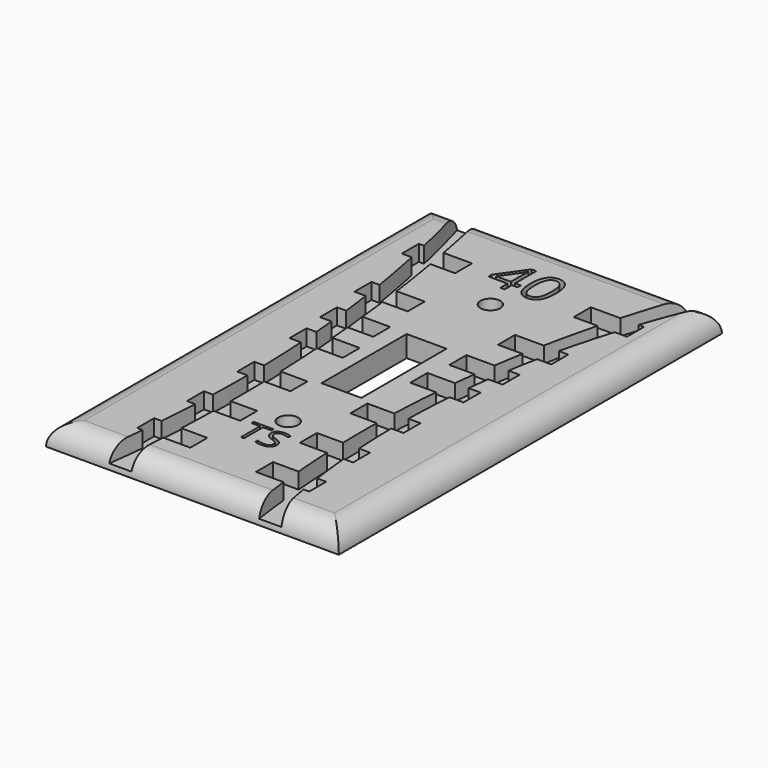
from build123d import *

# Parameters (mm, degrees)
F1_DEPTH     = 5.08
F4_R         = 5.07999
F2_TEXT_SIZE = 8.8219803325
F3_TEXT_SIZE = 13.1538772758
F5_DEPTH     = 3.81


# Not quite as in the source:
# - a fillet or chamfer is up to 0.001 mm smaller than in the source, because OpenCascade refuses the exact size
# - Text() gives the source's letters only with a copy of the font that has no kerning and outlines rounded to 1/6400 em; it was checked with that copy


with BuildPart() as f1:
    # F0 (on Top) → F1 (new body)
    with BuildSketch(Plane.XY):
        with BuildLine():
            Line((0, 34.13125), (0, 57.15))
            Line((0, 57.15), (-34.925, 57.15))
            Line((-34.925, 57.15), (-34.925, 0))
            Line((-34.925, 0), (-4.7625, 0))
            Line((-4.7625, 0), (-4.7625, 12.7))
            Line((-4.7625, 12.7), (0, 12.7))
            Line((0, 12.7), (0, 29.36875))
            ThreePointArc((0, 29.36875), (-2.38125, 31.75), (0, 34.13125))
        make_face()
        with BuildLine():
            Line((34.925, 57.15), (0, 57.15))
            Line((0, 57.15), (0, 34.13125))
            ThreePointArc((0, 34.13125), (1.6837980227, 33.4337980227), (2.38125, 31.75))
            ThreePointArc((2.38125, 31.75), (1.6837980227, 30.0662019773), (0, 29.36875))
            Line((0, 29.36875), (0, 12.7))
            Line((0, 12.7), (4.7625, 12.7))
            Line((4.7625, 12.7), (4.7625, 0))
            Line((4.7625, 0), (34.925, 0))
            Line((34.925, 0), (34.925, 57.15))
        make_face()
        with BuildLine():
            Line((-4.7625, 0), (-34.925, 0))
            Line((-34.925, 0), (-34.925, -57.15))
            Line((-34.925, -57.15), (0, -57.15))
            Line((0, -57.15), (0, -30.95625))
            ThreePointArc((0, -30.95625), (-2.38125, -28.575), (0, -26.19375))
            Line((0, -26.19375), (0, -12.7))
            Line((0, -12.7), (-4.7625, -12.7))
            Line((-4.7625, -12.7), (-4.7625, 0))
        make_face()
        with BuildLine():
            Line((34.925, -57.15), (34.925, 0))
            Line((34.925, 0), (4.7625, 0))
            Line((4.7625, 0), (4.7625, -12.7))
            Line((4.7625, -12.7), (0, -12.7))
            Line((0, -12.7), (0, -26.19375))
            ThreePointArc((0, -26.19375), (1.6837980227, -26.8912019773), (2.38125, -28.575))
            ThreePointArc((2.38125, -28.575), (1.6837980227, -30.2587980227), (0, -30.95625))
            Line((0, -30.95625), (0, -57.15))
            Line((0, -57.15), (34.925, -57.15))
        make_face()
    extrude(amount=F1_DEPTH)

    # F4 (radius 5.08 in the source; OpenCascade refuses exactly that, so slightly less here)
    f4_edges = [f1.edges().sort_by_distance(p)[0] for p in [
        (0, 57.15, 5.08),
        (-34.925, 0, 5.08),
        (34.925, 0, 5.08),
        (0, -57.15, 5.08),
    ]]
    fillet(f4_edges, radius=F4_R)

    # F2 (on face) + F3 (on face) → F5 (cut)
    with BuildSketch(Plane.XY.offset(5.08)):
        with BuildLine():
            Line((-18.9645993921, -48.2939412492), (-14.0614041805, -48.2939412492))
            ThreePointArc((-14.0614041805, -48.2939412492), (-13.9250653867, -45.754370655), (-13.8057946727, -43.2139412492))
            Line((-13.8057946727, -43.2139412492), (-18.4952719082, -43.2139412492))
            ThreePointArc((-18.4952719082, -43.2139412492), (-18.7184675008, -45.7550007605), (-18.9645993921, -48.2939412492))
        make_face()
        with BuildLine():
            ThreePointArc((-13.8057946727, -43.2139412492), (-13.9250653867, -45.754370655), (-14.0614041805, -48.2939412492))
            Line((-14.0614041805, -48.2939412492), (-7.5750437806, -48.2939412492))
            Line((-7.5750437806, -48.2939412492), (-7.5750437806, -43.2139412492))
            Line((-7.5750437806, -43.2139412492), (-13.8057946727, -43.2139412492))
        make_face()
        with BuildLine():
            Line((-18.4952719082, -43.2139412492), (-13.8057946727, -43.2139412492))
            ThreePointArc((-13.8057946727, -43.2139412492), (-13.6333233135, -38.6135289997), (-13.5168216221, -34.0113592298))
            Line((-13.5168216221, -34.0113592298), (-17.8798988895, -34.0113592298))
            ThreePointArc((-17.8798988895, -34.0113592298), (-18.1500251347, -38.6151618795), (-18.4952719082, -43.2139412492))
        make_face()
        with BuildLine():
            Line((-20.2750437806, -48.2939412492), (-18.9645993921, -48.2939412492))
            ThreePointArc((-18.9645993921, -48.2939412492), (-18.7184675008, -45.7550007605), (-18.4952719082, -43.2139412492))
            Line((-18.4952719082, -43.2139412492), (-20.2750437806, -43.2139412492))
            Line((-20.2750437806, -43.2139412492), (-20.2750437806, -48.2939412492))
        make_face()
        with BuildLine():
            Line((-17.8798988895, -34.0113592298), (-13.5168216221, -34.0113592298))
            ThreePointArc((-13.5168216221, -34.0113592298), (-13.4765066558, -31.4714659166), (-13.4532395385, -28.9313592298))
            Line((-13.4532395385, -28.9313592298), (-17.6692367261, -28.9313592298))
            ThreePointArc((-17.6692367261, -28.9313592298), (-17.7631384769, -31.4718331919), (-17.8798988895, -34.0113592298))
        make_face()
        with BuildLine():
            ThreePointArc((-13.4532395385, -28.9313592298), (-13.4765066558, -31.4714659166), (-13.5168216221, -34.0113592298))
            Line((-13.5168216221, -34.0113592298), (-7.1265053205, -34.0113592298))
            Line((-7.1265053205, -34.0113592298), (-7.1265053205, -28.9313592298))
            Line((-7.1265053205, -28.9313592298), (-13.4532395385, -28.9313592298))
        make_face()
        with BuildLine():
            Line((-17.6692367261, -28.9313592298), (-13.4532395385, -28.9313592298))
            ThreePointArc((-13.4532395385, -28.9313592298), (-13.4575297434, -23.8936067695), (-13.5288739929, -18.8563576934))
            Line((-13.5288739929, -18.8563576934), (-17.522028035, -18.8563576934))
            ThreePointArc((-17.522028035, -18.8563576934), (-17.5507079458, -23.8945148652), (-17.6692367261, -28.9313592298))
        make_face()
        with BuildLine():
            Line((-19.8265053205, -34.0113592298), (-17.8798988895, -34.0113592298))
            ThreePointArc((-17.8798988895, -34.0113592298), (-17.7631384769, -31.4718331919), (-17.6692367261, -28.9313592298))
            Line((-17.6692367261, -28.9313592298), (-19.8265053205, -28.9313592298))
            Line((-19.8265053205, -28.9313592298), (-19.8265053205, -34.0113592298))
        make_face()
        with BuildLine():
            Line((-17.522028035, -18.8563576934), (-13.5288739929, -18.8563576934))
            ThreePointArc((-13.5288739929, -18.8563576934), (-13.5902952465, -16.3161228869), (-13.6687694767, -13.7763576934))
            Line((-13.6687694767, -13.7763576934), (-17.5840967399, -13.7763576934))
            ThreePointArc((-17.5840967399, -13.7763576934), (-17.5416420192, -16.3162181565), (-17.522028035, -18.8563576934))
        make_face()
        with BuildLine():
            ThreePointArc((-13.6687694767, -13.7763576934), (-13.5902952465, -16.3161228869), (-13.5288739929, -18.8563576934))
            Line((-13.5288739929, -18.8563576934), (-7.2402887804, -18.8563576934))
            Line((-7.2402887804, -18.8563576934), (-7.2402887804, -13.7763576934))
            Line((-7.2402887804, -13.7763576934), (-13.6687694767, -13.7763576934))
        make_face()
        with BuildLine():
            Line((-17.5840967399, -13.7763576934), (-13.6687694767, -13.7763576934))
            ThreePointArc((-13.6687694767, -13.7763576934), (-13.910836625, -8.0001298482), (-14.2411063378, -2.2282734276))
            Line((-14.2411063378, -2.2282734276), (-18.0655749495, -2.2282734276))
            ThreePointArc((-18.0655749495, -2.2282734276), (-17.765767613, -7.9998528086), (-17.5840967399, -13.7763576934))
        make_face()
        with BuildLine():
            Line((-19.9402887804, -18.8563576934), (-17.522028035, -18.8563576934))
            ThreePointArc((-17.522028035, -18.8563576934), (-17.5416420192, -16.3162181565), (-17.5840967399, -13.7763576934))
            Line((-17.5840967399, -13.7763576934), (-19.9402887804, -13.7763576934))
            Line((-19.9402887804, -13.7763576934), (-19.9402887804, -18.8563576934))
        make_face()
        with BuildLine():
            Line((-18.0655749495, -2.2282734276), (-14.2411063378, -2.2282734276))
            ThreePointArc((-14.2411063378, -2.2282734276), (-14.4145438637, 0.3123388011), (-14.6050716004, 2.8517265724))
            Line((-14.6050716004, 2.8517265724), (-18.4275918721, 2.8517265724))
            ThreePointArc((-18.4275918721, 2.8517265725), (-18.2351349339, 0.3125424272), (-18.0655749495, -2.2282734276))
        make_face()
        with BuildLine():
            ThreePointArc((-14.6050716004, 2.8517265724), (-14.4145438637, 0.3123388011), (-14.2411063378, -2.2282734276))
            Line((-14.2411063378, -2.2282734276), (-8.0645, -2.2282734276))
            Line((-8.0645, -2.2282734276), (-8.0645, 2.8517265724))
            Line((-8.0645, 2.8517265724), (-14.6050716004, 2.8517265724))
        make_face()
        with BuildLine():
            Line((-18.4275918721, 2.8517265724), (-14.6050716004, 2.8517265724))
            ThreePointArc((-14.6050716004, 2.8517265724), (-14.8129092664, 5.39245533), (-15.0378551973, 7.9317265724))
            Line((-15.0378551973, 7.9317265724), (-18.8818564891, 7.9317265724))
            ThreePointArc((-18.8818564891, 7.9317265724), (-18.6432590968, 5.3927518051), (-18.4275918721, 2.8517265725))
        make_face()
        with BuildLine():
            Line((-20.7645, -2.2282734276), (-18.0655749495, -2.2282734276))
            ThreePointArc((-18.0655749495, -2.2282734276), (-18.2351349339, 0.3125424272), (-18.4275918721, 2.8517265725))
            Line((-18.4275918721, 2.8517265724), (-20.7645, 2.8517265724))
            Line((-20.7645, 2.8517265724), (-20.7645, -2.2282734276))
        make_face()
        with BuildLine():
            Line((-18.8818564891, 7.9317265724), (-15.0378551973, 7.9317265724))
            ThreePointArc((-15.0378551973, 7.9317265724), (-15.2802101133, 10.4725726603), (-15.539694521, 13.0117265725))
            Line((-15.539694521, 13.0117265724), (-19.4288168547, 13.0117265724))
            ThreePointArc((-19.4288168547, 13.0117265725), (-19.1438511527, 10.472963211), (-18.8818564891, 7.9317265724))
        make_face()
        with BuildLine():
            ThreePointArc((-15.539694521, 13.0117265725), (-15.2802101133, 10.4725726603), (-15.0378551973, 7.9317265724))
            Line((-15.0378551973, 7.9317265724), (-8.9301265316, 7.9317265724))
            Line((-8.9301265316, 7.9317265724), (-8.9301265316, 13.0117265724))
            Line((-8.9301265316, 13.0117265724), (-15.539694521, 13.0117265724))
        make_face()
        with BuildLine():
            Line((-19.4288168547, 13.0117265724), (-15.539694521, 13.0117265724))
            ThreePointArc((-15.539694521, 13.0117265725), (-15.9227086621, 16.4850893922), (-16.3377753353, 19.9547678739))
            Line((-16.3377753353, 19.9547678739), (-20.3272945329, 19.9547678739))
            ThreePointArc((-20.3272945328, 19.9547678739), (-19.8565460149, 16.4860307247), (-19.4288168547, 13.0117265725))
        make_face()
        with BuildLine():
            Line((-21.6301265316, 7.9317265724), (-18.8818564891, 7.9317265724))
            ThreePointArc((-18.8818564891, 7.9317265724), (-19.1438511527, 10.472963211), (-19.4288168547, 13.0117265725))
            Line((-19.4288168547, 13.0117265724), (-21.6301265316, 13.0117265724))
            Line((-21.6301265316, 13.0117265724), (-21.6301265316, 7.9317265724))
        make_face()
        with BuildLine():
            Line((-20.3272945329, 19.9547678739), (-16.3377753353, 19.9547678739))
            ThreePointArc((-16.3377753353, 19.9547678739), (-16.6624046702, 22.4958956318), (-17.0042265914, 25.0347678739))
            Line((-17.0042265914, 25.0347678739), (-21.0959848739, 25.0347678739))
            ThreePointArc((-21.0959848739, 25.0347678739), (-20.7000901868, 22.4965155121), (-20.3272945328, 19.9547678739))
        make_face()
        with BuildLine():
            ThreePointArc((-17.0042265914, 25.0347678739), (-16.6624046702, 22.4958956318), (-16.3377753353, 19.9547678739))
            Line((-16.3377753353, 19.9547678739), (-10.31225672, 19.9547678739))
            Line((-10.31225672, 19.9547678739), (-10.31225672, 25.0347678739))
            Line((-10.31225672, 25.0347678739), (-17.0042265914, 25.0347678739))
        make_face()
        with BuildLine():
            Line((-21.0959848739, 25.0347678739), (-17.0042265914, 25.0347678739))
            ThreePointArc((-17.0042265914, 25.0347678739), (-17.9183733157, 31.2713322394), (-18.936254879, 37.4918078193))
            Line((-18.936254879, 37.4918078193), (-23.3845623231, 37.4918078193))
            ThreePointArc((-23.3845623231, 37.4918078193), (-22.1704497166, 31.2761157225), (-21.0959848739, 25.0347678739))
        make_face()
        with BuildLine():
            Line((-23.01225672, 19.9547678739), (-20.3272945329, 19.9547678739))
            ThreePointArc((-20.3272945328, 19.9547678739), (-20.7000901868, 22.4965155121), (-21.0959848739, 25.0347678739))
            Line((-21.0959848739, 25.0347678739), (-23.01225672, 25.0347678739))
            Line((-23.01225672, 25.0347678739), (-23.01225672, 19.9547678739))
        make_face()
        with BuildLine():
            Line((-23.3845623231, 37.4918078193), (-18.936254879, 37.4918078193))
            ThreePointArc((-18.936254879, 37.4918078193), (-19.3828266958, 40.0333597387), (-19.8467166487, 42.5718078193))
            Line((-19.8467166487, 42.5718078193), (-24.4849250128, 42.5718078193))
            ThreePointArc((-24.4849250128, 42.5718078193), (-23.9230593184, 40.0343387292), (-23.3845623231, 37.4918078193))
        make_face()
        with BuildLine():
            ThreePointArc((-19.8467166487, 42.5718078193), (-19.3828266958, 40.0333597387), (-18.936254879, 37.4918078193))
            Line((-18.936254879, 37.4918078193), (-13.0325485568, 37.4918078193))
            Line((-13.0325485568, 37.4918078193), (-13.0325485568, 42.5718078193))
            Line((-13.0325485568, 42.5718078193), (-19.8467166487, 42.5718078193))
        make_face()
        with BuildLine():
            Line((-25.7325485568, 37.4918078193), (-23.3845623231, 37.4918078193))
            ThreePointArc((-23.3845623231, 37.4918078193), (-23.9230593184, 40.0343387292), (-24.4849250128, 42.5718078193))
            Line((-24.4849250128, 42.5718078193), (-25.7325485568, 42.5718078193))
            Line((-25.7325485568, 42.5718078193), (-25.7325485568, 37.4918078193))
        make_face()
        with BuildLine():
            Line((26.6740367785, 42.5718078193), (22.3445437559, 42.5718078193))
            ThreePointArc((22.3445437559, 42.5718078193), (21.6434222097, 40.0355750124), (20.9701490551, 37.4918078193))
            Line((20.9701490551, 37.4918078193), (25.0346873706, 37.4918078193))
            ThreePointArc((25.0346873706, 37.4918078193), (25.8361879773, 40.03767272), (26.6740367785, 42.5718078193))
        make_face()
        with BuildLine():
            ThreePointArc((20.9701490551, 37.4918078193), (21.6434222097, 40.0355750124), (22.3445437559, 42.5718078193))
            Line((22.3445437559, 42.5718078193), (15.292403028, 42.5718078193))
            Line((15.292403028, 42.5718078193), (15.292403028, 37.4918078193))
            Line((15.292403028, 37.4918078193), (20.9701490551, 37.4918078193))
        make_face()
        with BuildLine():
            Line((25.0346873706, 37.4918078193), (20.9701490551, 37.4918078193))
            ThreePointArc((20.9701490551, 37.4918078193), (19.4509835882, 31.2824162557), (18.0977293612, 25.0347678739))
            Line((18.0977293612, 25.0347678739), (21.6774065425, 25.0347678739))
            ThreePointArc((21.6774065425, 25.0347678739), (23.2483069936, 31.2923247056), (25.0346873706, 37.4918078193))
        make_face()
        with BuildLine():
            Line((27.992403028, 42.5718078193), (26.6740367785, 42.5718078193))
            ThreePointArc((26.6740367785, 42.5718078193), (25.8361879773, 40.03767272), (25.0346873706, 37.4918078193))
            Line((25.0346873706, 37.4918078193), (27.992403028, 37.4918078193))
            Line((27.992403028, 37.4918078193), (27.992403028, 42.5718078193))
        make_face()
        with BuildLine():
            Line((21.6774065425, 25.0347678739), (18.0977293612, 25.0347678739))
            ThreePointArc((18.0977293612, 25.0347678739), (17.5976230219, 22.4973886486), (17.1248870709, 19.9547678739))
            Line((17.1248870709, 19.9547678739), (20.569534352, 19.9547678739))
            ThreePointArc((20.569534352, 19.9547678739), (21.105768159, 22.4986284788), (21.6774065425, 25.0347678739))
        make_face()
        with BuildLine():
            ThreePointArc((17.1248870709, 19.9547678739), (17.5976230219, 22.4973886486), (18.0977293612, 25.0347678739))
            Line((18.0977293612, 25.0347678739), (11.2471211472, 25.0347678739))
            Line((11.2471211472, 25.0347678739), (11.2471211472, 19.9547678739))
            Line((11.2471211472, 19.9547678739), (17.1248870709, 19.9547678739))
        make_face()
        with BuildLine():
            Line((20.569534352, 19.9547678739), (17.1248870709, 19.9547678739))
            ThreePointArc((17.1248870709, 19.9547678739), (16.525745384, 16.4874526893), (15.9775008428, 13.0117263949))
            Line((15.9775008428, 13.0117263949), (19.2927738954, 13.0117263949))
            ThreePointArc((19.2927738954, 13.0117263949), (19.898302927, 16.4892881625), (20.569534352, 19.9547678739))
        make_face()
        with BuildLine():
            Line((23.9471211472, 25.0347678739), (21.6774065425, 25.0347678739))
            ThreePointArc((21.6774065425, 25.0347678739), (21.105768159, 22.4986284788), (20.569534352, 19.9547678739))
            Line((20.569534352, 19.9547678739), (23.9471211472, 19.9547678739))
            Line((23.9471211472, 19.9547678739), (23.9471211472, 25.0347678739))
        make_face()
        with BuildLine():
            Line((19.2927738954, 13.0117263949), (15.9775008428, 13.0117263949))
            ThreePointArc((15.9775008428, 13.0117263949), (15.610054084, 10.4736170904), (15.2697488468, 7.9317263949))
            Line((15.2697488468, 7.9317263949), (18.5293608453, 7.9317263949))
            ThreePointArc((18.5293608453, 7.9317263949), (18.8935774183, 10.4743547527), (19.2927738954, 13.0117263949))
        make_face()
        with BuildLine():
            ThreePointArc((15.2697488468, 7.9317263949), (15.610054084, 10.4736170904), (15.9775008428, 13.0117263949))
            Line((15.9775008428, 13.0117263949), (9.2597906775, 13.0117263949))
            Line((9.2597906775, 13.0117263949), (9.2597906775, 7.9317263949))
            Line((9.2597906775, 7.9317263949), (15.2697488468, 7.9317263949))
        make_face()
        with BuildLine():
            Line((18.5293608453, 7.9317263949), (15.2697488468, 7.9317263949))
            ThreePointArc((15.2697488468, 7.9317263949), (14.9574441825, 5.393318304), (14.672206725, 2.8517263949))
            Line((14.672206725, 2.8517263949), (17.9082056584, 2.8517263949))
            ThreePointArc((17.9082056584, 2.8517263949), (18.2013586996, 5.3938569758), (18.5293608453, 7.9317263949))
        make_face()
        with BuildLine():
            Line((21.9597906775, 13.0117263949), (19.2927738954, 13.0117263949))
            ThreePointArc((19.2927738954, 13.0117263949), (18.8935774183, 10.4743547527), (18.5293608453, 7.9317263949))
            Line((18.5293608453, 7.9317263949), (21.9597906775, 7.9317263949))
            Line((21.9597906775, 7.9317263949), (21.9597906775, 13.0117263949))
        make_face()
        with BuildLine():
            Line((17.9082056584, 2.8517263949), (14.672206725, 2.8517263949))
            ThreePointArc((14.672206725, 2.8517263949), (14.414624683, 0.3130241177), (14.1840483405, -2.22827325))
            Line((14.1840483405, -2.22827325), (17.4278824523, -2.22827325))
            ThreePointArc((17.4278824523, -2.22827325), (17.6506711854, 0.3133692089), (17.9082056584, 2.8517263949))
        make_face()
        with BuildLine():
            ThreePointArc((14.1840483405, -2.22827325), (14.414624683, 0.3130241177), (14.672206725, 2.8517263949))
            Line((14.672206725, 2.8517263949), (8.0645, 2.8517263949))
            Line((8.0645, 2.8517263949), (8.0645, -2.22827325))
            Line((8.0645, -2.22827325), (14.1840483405, -2.22827325))
        make_face()
        with BuildLine():
            Line((17.4278824523, -2.22827325), (14.1840483405, -2.22827325))
            ThreePointArc((14.1840483405, -2.22827325), (13.7614351398, -7.9980604756), (13.4780135303, -13.7763576934))
            Line((13.4780135303, -13.7763576934), (16.8547186556, -13.7763576934))
            ThreePointArc((16.8547186556, -13.7763576934), (17.0517950543, -7.9978730629), (17.4278824523, -2.22827325))
        make_face()
        with BuildLine():
            Line((20.7645, 2.8517263949), (17.9082056584, 2.8517263949))
            ThreePointArc((17.9082056584, 2.8517263949), (17.6506711854, 0.3133692089), (17.4278824523, -2.22827325))
            Line((17.4278824523, -2.22827325), (20.7645, -2.22827325))
            Line((20.7645, -2.22827325), (20.7645, 2.8517263949))
        make_face()
        with BuildLine():
            Line((16.8547186556, -13.7763576934), (13.4780135303, -13.7763576934))
            ThreePointArc((13.4780135303, -13.7763576934), (13.3975715183, -16.3160030449), (13.3440207231, -18.8563576934))
            Line((13.3440207231, -18.8563576934), (16.829454419, -18.8563576934))
            ThreePointArc((16.829454419, -18.8563576934), (16.8247905984, -16.316271676), (16.8547186556, -13.7763576934))
        make_face()
        with BuildLine():
            ThreePointArc((13.3440207231, -18.8563576934), (13.3975715183, -16.3160030449), (13.4780135303, -13.7763576934))
            Line((13.4780135303, -13.7763576934), (7.0475621641, -13.7763576934))
            Line((7.0475621641, -13.7763576934), (7.0475621641, -18.8563576934))
            Line((7.0475621641, -18.8563576934), (13.3440207231, -18.8563576934))
        make_face()
        with BuildLine():
            Line((16.829454419, -18.8563576934), (13.3440207231, -18.8563576934))
            ThreePointArc((13.3440207231, -18.8563576934), (13.3173810289, -23.894133803), (13.3964873009, -28.9313592298))
            Line((13.3964873009, -28.9313592298), (17.1890239139, -28.9313592298))
            ThreePointArc((17.1890239139, -28.9313592298), (16.941156402, -23.8962882861), (16.829454419, -18.8563576934))
        make_face()
        with BuildLine():
            Line((19.7475621641, -13.7763576934), (16.8547186556, -13.7763576934))
            ThreePointArc((16.8547186556, -13.7763576934), (16.8247905984, -16.316271676), (16.829454419, -18.8563576934))
            Line((16.829454419, -18.8563576934), (19.7475621641, -18.8563576934))
            Line((19.7475621641, -18.8563576934), (19.7475621641, -13.7763576934))
        make_face()
        with BuildLine():
            Line((17.1890239139, -28.9313592298), (13.3964873009, -28.9313592298))
            ThreePointArc((13.3964873009, -28.9313592298), (13.4765235401, -31.4718542667), (13.5834598487, -34.0113592298))
            Line((13.5834598487, -34.0113592298), (17.577694227, -34.0113592298))
            ThreePointArc((17.577694227, -34.0113592298), (17.3660127922, -31.4726863919), (17.1890239139, -28.9313592298))
        make_face()
        with BuildLine():
            ThreePointArc((13.5834598487, -34.0113592298), (13.4765235401, -31.4718542667), (13.3964873009, -28.9313592298))
            Line((13.3964873009, -28.9313592298), (7.1265053205, -28.9313592298))
            Line((7.1265053205, -28.9313592298), (7.1265053205, -34.0113592298))
            Line((7.1265053205, -34.0113592298), (13.5834598487, -34.0113592298))
        make_face()
        with BuildLine():
            Line((17.577694227, -34.0113592298), (13.5834598487, -34.0113592298))
            ThreePointArc((13.5834598487, -34.0113592298), (13.8461269924, -38.6155987103), (14.1972126185, -43.2139412492))
            Line((14.1972126185, -43.2139412492), (18.6393301719, -43.2139412492))
            ThreePointArc((18.6393301719, -43.2139412492), (18.0513711209, -38.6192421963), (17.577694227, -34.0113592298))
        make_face()
        with BuildLine():
            Line((19.8265053205, -28.9313592298), (17.1890239139, -28.9313592298))
            ThreePointArc((17.1890239139, -28.9313592298), (17.3660127922, -31.4726863919), (17.577694227, -34.0113592298))
            Line((17.577694227, -34.0113592298), (19.8265053205, -34.0113592298))
            Line((19.8265053205, -34.0113592298), (19.8265053205, -28.9313592298))
        make_face()
        with BuildLine():
            Line((18.6393301719, -43.2139412492), (14.1972126185, -43.2139412492))
            ThreePointArc((14.1972126185, -43.2139412492), (14.4294366561, -45.7552476392), (14.6886680716, -48.2939412492))
            Line((14.6886680716, -48.2939412492), (19.4251434202, -48.2939412492))
            ThreePointArc((19.4251434202, -48.2939412492), (19.0147353466, -45.7566485072), (18.6393301719, -43.2139412492))
        make_face()
        with BuildLine():
            ThreePointArc((14.6886680716, -48.2939412492), (14.4294366561, -45.7552476392), (14.1972126185, -43.2139412492))
            Line((14.1972126185, -43.2139412492), (8.0793102754, -43.2139412492))
            Line((8.0793102754, -43.2139412492), (8.0793102754, -48.2939412492))
            Line((8.0793102754, -48.2939412492), (14.6886680716, -48.2939412492))
        make_face()
        with BuildLine():
            Line((20.7793102754, -43.2139412492), (18.6393301719, -43.2139412492))
            ThreePointArc((18.6393301719, -43.2139412492), (19.0147353466, -45.7566485072), (19.4251434202, -48.2939412492))
            Line((19.4251434202, -48.2939412492), (20.7793102754, -48.2939412492))
            Line((20.7793102754, -48.2939412492), (20.7793102754, -43.2139412492))
        make_face()
        with Locations((-4.9361736829, -39.07708736)):
            Text('TS', F2_TEXT_SIZE, font='Open Sans', text_align=(TextAlign.LEFT, TextAlign.BOTTOM))
        with BuildLine():
            Line((-20.0049679099, -57.15), (-14.6709679099, -57.15))
            ThreePointArc((-14.6709679099, -57.15), (-14.3402206162, -52.7237578286), (-14.0614041805, -48.2939412492))
            Line((-14.0614041805, -48.2939412492), (-18.9645993921, -48.2939412492))
            ThreePointArc((-18.9645993921, -48.2939412492), (-19.4498377893, -52.7260759016), (-20.0049679099, -57.15))
        make_face()
        with BuildLine():
            Line((-22.86, 57.15), (-28.194, 57.15))
            ThreePointArc((-28.194, 57.15), (-26.2424079074, 49.8855971488), (-24.4849250128, 42.5718078193))
            Line((-24.4849250128, 42.5718078193), (-19.8467166487, 42.5718078193))
            ThreePointArc((-19.8467166487, 42.5718078193), (-21.2816767879, 49.8757203408), (-22.86, 57.15))
        make_face()
        with BuildLine():
            ThreePointArc((14.6886680716, -48.2939412492), (15.2069250238, -52.7271727974), (15.8075345178, -57.15))
            Line((15.8075345178, -57.15), (21.1415345178, -57.15))
            ThreePointArc((21.1415345178, -57.15), (20.2297910285, -52.732348741), (19.4251434202, -48.2939412492))
            Line((19.4251434202, -48.2939412492), (14.6886680716, -48.2939412492))
        make_face()
        with BuildLine():
            ThreePointArc((26.6740367785, 42.5718078193), (29.3347999027, 49.9198588288), (32.3010387137, 57.15))
            Line((32.3010387137, 57.15), (26.9670387137, 57.15))
            ThreePointArc((26.9670387137, 57.15), (24.5396435221, 49.8977323593), (22.3445437559, 42.5718078193))
            Line((22.3445437559, 42.5718078193), (26.6740367785, 42.5718078193))
        make_face()
    with BuildSketch(Plane.XY.offset(5.08)):
        with Locations((-7.62, 38.1898654068)):
            Text('40', F3_TEXT_SIZE, font='Open Sans', text_align=(TextAlign.LEFT, TextAlign.BOTTOM))
    extrude(amount=-F5_DEPTH, mode=Mode.SUBTRACT)


solid = f1.part
